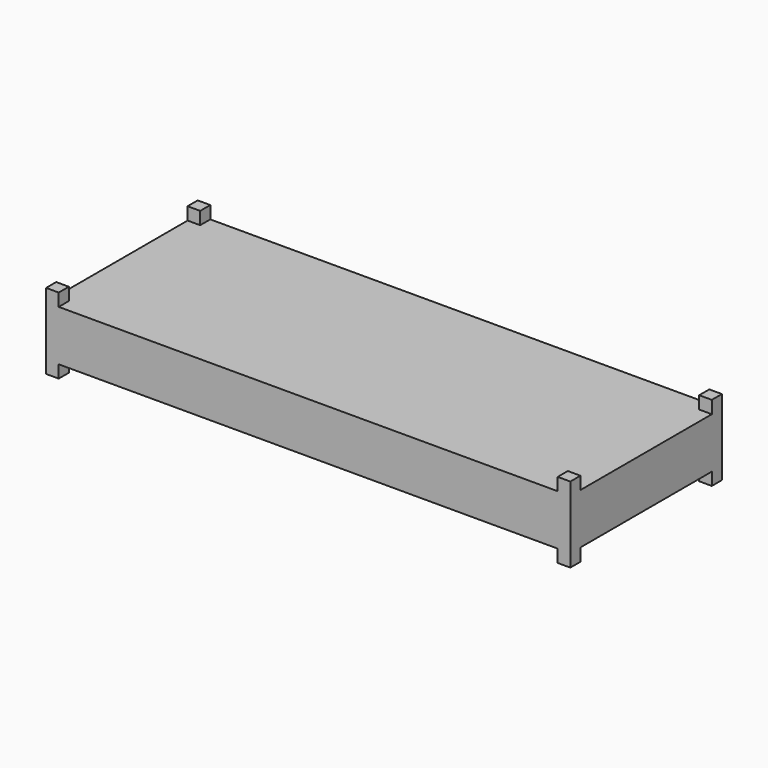
from build123d import *

# Parameters (mm, degrees)
F0_W     = 527.05
F0_H     = 190.5
F1_DEPTH = 38.1
F3_DEPTH = 12.7


# Not quite as in the source:
# - a pattern or mirror of a feature is missing from the dataset's text; its kind, count and spacing are read off the source's solid


with BuildPart() as f1:
    # F0 (on Top) → F1 (new body, symmetric)
    with BuildSketch(Plane.XY):
        Rectangle(F0_W, F0_H)
    extrude(amount=F1_DEPTH, both=True)

    # F2 (on face) → F3 (cut)
    with BuildSketch(Plane(origin=(0, 0, -38.1), x_dir=(1, 0, 0), z_dir=(0, 0, -1))):
        Polygon((250.825, 95.25), (-250.825, 95.25), (-250.825, 82.55), (-263.525, 82.55), (-263.525, -82.55), (-250.825, -82.55), (-250.825, -95.25), (250.825, -95.25), (250.825, -82.55), (263.525, -82.55), (263.525, 82.55), (250.825, 82.55), align=None)
    f3 = extrude(amount=-F3_DEPTH, mode=Mode.SUBTRACT)

    # F3_copies: F3 across plane
    add(f3.mirror(Plane.XY), mode=Mode.SUBTRACT)


solid = f1.part
